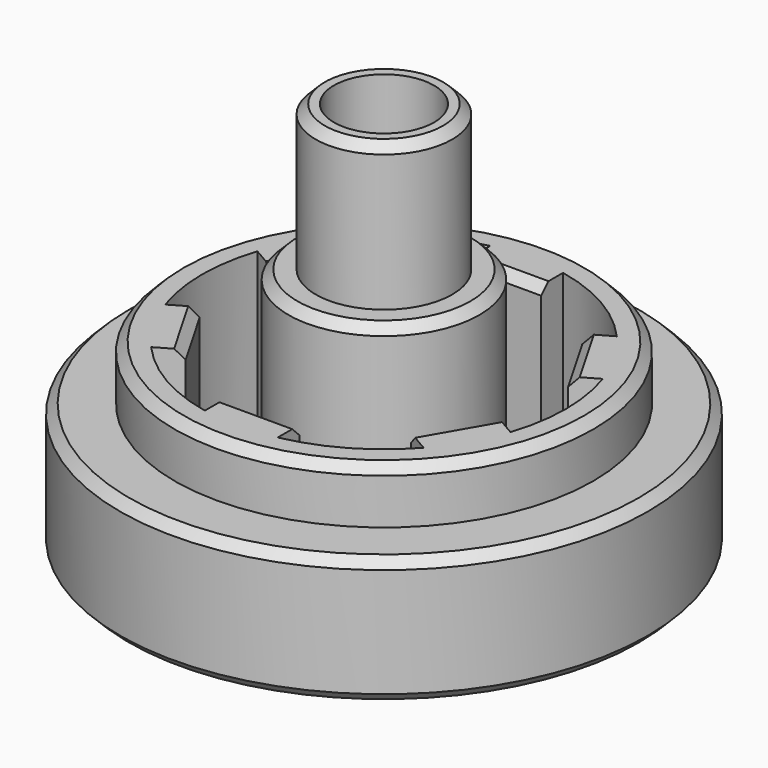
from build123d import *

# Parameters (mm, degrees)
F0_R      = 14.5
F1_DEPTH  = 10
F2_R      = 11.5
F3_DEPTH  = 9
F4_SIZE   = 0.5
F5_R      = 5.25
F6_DEPTH  = 12.5
F7_SIZE   = 0.5
F8_R      = 3.75
F9_DEPTH  = 8
F10_SIZE  = 0.5
F11_R     = 14.5
F11_R_2   = 11.5
F12_DEPTH = 6
F13_R     = 25
F14_DEPTH = 9
F15_SIZE  = 0.5
F16_R     = 2.75
F17_DEPTH = 19


with BuildPart() as f1:
    # F0 (on Top) → F1 (new body)
    with BuildSketch(Plane.XY):
        Circle(F0_R)
    extrude(amount=F1_DEPTH)

    # F2 (on face) → F3 (join)
    with BuildSketch(Plane.XY.offset(10)):
        Circle(F2_R)
        with BuildLine():
            ThreePointArc((-7.4852813742, 6.6310302931), (-5, 8.6602540378), (-2, 9.7979589711))
            Line((-2, 9.7979589711), (-2, 8.3))
            Line((-2, 8.3), (2, 8.3))
            Line((2, 8.3), (2, 9.7979589711))
            ThreePointArc((2, 9.7979589711), (5, 8.6602540378), (7.4852813742, 6.6310302931))
            Line((7.4852813742, 6.6310302931), (6.1880108514, 5.8820508076))
            Line((6.1880108514, 5.8820508076), (8.1880108514, 2.4179491924))
            Line((8.1880108514, 2.4179491924), (9.4852813742, 3.166928678))
            ThreePointArc((9.4852813742, 3.166928678), (10, 0), (9.4852813742, -3.166928678))
            Line((9.4852813742, -3.166928678), (8.1880108514, -2.4179491924))
            Line((8.1880108514, -2.4179491924), (6.1880108514, -5.8820508076))
            Line((6.1880108514, -5.8820508076), (7.4852813742, -6.6310302931))
            ThreePointArc((7.4852813742, -6.6310302931), (5, -8.6602540378), (2, -9.7979589711))
            Line((2, -9.7979589711), (2, -8.3))
            Line((2, -8.3), (-2, -8.3))
            Line((-2, -8.3), (-2, -9.7979589711))
            ThreePointArc((-2, -9.7979589711), (-5, -8.6602540378), (-7.4852813742, -6.6310302931))
            Line((-7.4852813742, -6.6310302931), (-6.1880108514, -5.8820508076))
            Line((-6.1880108514, -5.8820508076), (-8.1880108514, -2.4179491924))
            Line((-8.1880108514, -2.4179491924), (-9.4852813742, -3.166928678))
            ThreePointArc((-9.4852813742, -3.166928678), (-10, 0), (-9.4852813742, 3.166928678))
            Line((-9.4852813742, 3.166928678), (-8.1880108514, 2.4179491924))
            Line((-8.1880108514, 2.4179491924), (-6.1880108514, 5.8820508076))
            Line((-6.1880108514, 5.8820508076), (-7.4852813742, 6.6310302931))
        make_face(mode=Mode.SUBTRACT)
    extrude(amount=F3_DEPTH)

    # F4
    f4_edges = [f1.edges().sort_by_distance(p)[0] for p in [
        (0, 8.3, 19),
        (-7.188011, 4.15, 19),
        (-7.188011, -4.15, 19),
        (0, -8.3, 19),
        (7.188011, -4.15, 19),
        (7.188011, 4.15, 19),
    ]]
    chamfer(f4_edges, length=F4_SIZE)

    # F5 (on face) → F6 (join)
    with BuildSketch(Plane.XY.offset(10)):
        Circle(F5_R)
    extrude(amount=F6_DEPTH)

    # F7
    f7_edges = [f1.edges().sort_by_distance(p)[0] for p in [
        (-5.25, 0, 22.5),
    ]]
    chamfer(f7_edges, length=F7_SIZE)

    # F8 (on face) → F9 (join)
    with BuildSketch(Plane.XY.offset(22.5)):
        Circle(F8_R)
    extrude(amount=F9_DEPTH)

    # F10
    f10_edges = [f1.edges().sort_by_distance(p)[0] for p in [
        (-3.75, 0, 30.5),
    ]]
    chamfer(f10_edges, length=F10_SIZE)

    # F11 (on face) → F12 (join)
    with BuildSketch(Plane.XY.offset(10)):
        Circle(F11_R)
        Circle(F11_R_2, mode=Mode.SUBTRACT)
    extrude(amount=F12_DEPTH)

    # F13 (on face) → F14 (cut)
    with BuildSketch(Plane(origin=(0, 0, 0), x_dir=(1, 0, 0), z_dir=(0, 0, -1))):
        Circle(F13_R)
    extrude(amount=-F14_DEPTH, mode=Mode.SUBTRACT)

    # F15
    f15_edges = [f1.edges().sort_by_distance(p)[0] for p in [
        (-11.5, 0, 19),
        (-14.5, 0, 16),
        (-14.5, 0, 9),
    ]]
    chamfer(f15_edges, length=F15_SIZE)

    # F16 (on face) → F17 (cut)
    with BuildSketch(Plane.XY.offset(30.5)):
        Circle(F16_R)
    extrude(amount=-F17_DEPTH, mode=Mode.SUBTRACT)


solid = f1.part
